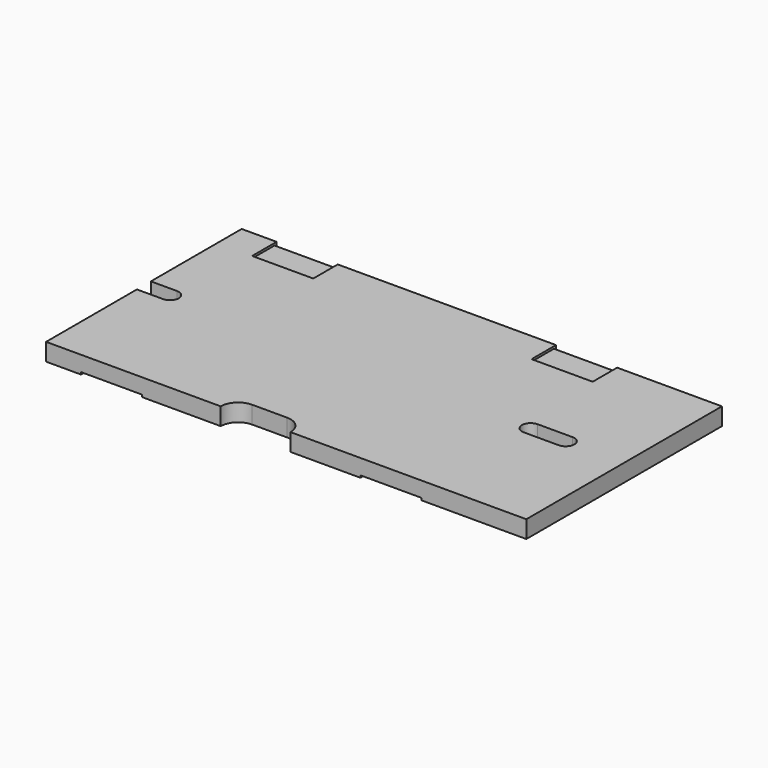
from build123d import *

# Parameters (mm, degrees)
F0_W      = 698.5
F0_H      = 355.6
F1_DEPTH  = 25.4
F2_W      = 88.9
F2_H      = 44.45
F3_DEPTH  = 3.175
F4_W      = 88.9
F4_H      = 44.45
F5_DEPTH  = 3.175
F6_W      = 88.9
F6_H      = 3.81
F7_DEPTH  = 3.175
F8_W      = 88.9
F8_H      = 3.81
F9_DEPTH  = 3.81
F11_DEPTH = 25.4
F12_W     = 101.6
F12_H     = 25.4
F13_DEPTH = 25.4
F14_R     = 25.39999


# Not quite as in the source:
# - a fillet or chamfer is up to 0.001 mm smaller than in the source, because OpenCascade refuses the exact size


with BuildPart() as f1:
    # F0 (on Top) → F1 (new body)
    with BuildSketch(Plane.XY):
        Rectangle(F0_W, F0_H)
    extrude(amount=F1_DEPTH)

    # F2 (on face) → F3 (cut)
    with BuildSketch(Plane.XY.offset(25.4)):
        with Locations((-254, 155.575)):
            Rectangle(F2_W, F2_H)
        with Locations((152.4, 155.575)):
            Rectangle(F2_W, F2_H)
    extrude(amount=-F3_DEPTH, mode=Mode.SUBTRACT)

    # F4 (on face) → F5 (cut)
    with BuildSketch(Plane(origin=(0, 0, 0), x_dir=(1, 0, 0), z_dir=(0, 0, -1))):
        with Locations((-254, 155.575)):
            Rectangle(F4_W, F4_H)
        with Locations((152.4, 155.575)):
            Rectangle(F4_W, F4_H)
    extrude(amount=-F5_DEPTH, mode=Mode.SUBTRACT)

    # F6 (on face) → F7 (cut)
    with BuildSketch(Plane.XY.offset(22.225)):
        with Locations((-254, 175.895)):
            Rectangle(F6_W, F6_H)
    extrude(amount=-F7_DEPTH, mode=Mode.SUBTRACT)

    # F8 (on face) → F9 (cut)
    with BuildSketch(Plane.XY.offset(22.225)):
        with Locations((152.4, 175.895)):
            Rectangle(F8_W, F8_H)
    extrude(amount=-F9_DEPTH, mode=Mode.SUBTRACT)

    # F10 (on face) → F11 (cut)
    with BuildSketch(Plane.XY.offset(25.4)):
        with BuildLine():
            Line((-311.0040204385, -12.7008390054), (-311.0040204385, -12.6991609946))
            ThreePointArc((-311.0040204385, -12.6991609946), (-298.45, 0), (-311.0040204385, 12.6991609946))
            Line((-311.0040204385, 12.6991609946), (-311.2959795615, 12.6991609946))
            Line((-311.2959795615, 12.6991609946), (-354.8822260717, 12.6991609946))
            Line((-354.8822260717, 12.6991609946), (-354.8822260717, -12.7008390054))
            Line((-354.8822260717, -12.7008390054), (-311.0040204385, -12.7008390054))
        make_face()
        with BuildLine():
            Line((-311.2959795615, 12.6991609946), (-311.0040204385, 12.6991609946))
            ThreePointArc((-311.0040204385, 12.6991609946), (-311.15, 12.7), (-311.2959795615, 12.6991609946))
        make_face()
        with BuildLine():
            Line((213.1756003467, 12.7013387805), (213.1756003467, 12.6986612195))
            ThreePointArc((213.1756003467, 12.6986612195), (200.66, 0), (213.1756003467, -12.6986612195))
            Line((213.1756003467, -12.6986612195), (213.5443996533, -12.6986612195))
            Line((213.5443996533, -12.6986612195), (264.16, -12.6986612195))
            ThreePointArc((264.16, -12.6986612195), (276.86, 0.0013387805), (264.16, 12.7013387805))
            Line((264.16, 12.7013387805), (213.1756003467, 12.7013387805))
        make_face()
        with BuildLine():
            Line((213.5443996533, -12.6986612195), (213.1756003467, -12.6986612195))
            ThreePointArc((213.1756003467, -12.6986612195), (213.36, -12.7), (213.5443996533, -12.6986612195))
        make_face()
    extrude(amount=-F11_DEPTH, mode=Mode.SUBTRACT)

    # F12 (on face) → F13 (cut)
    with BuildSketch(Plane.XY.offset(25.4)):
        with Locations((-44.45, -165.1)):
            Rectangle(F12_W, F12_H)
    extrude(amount=-F13_DEPTH, mode=Mode.SUBTRACT)

    # F14 (radius 25.4 in the source; OpenCascade refuses exactly that, so slightly less here)
    f14_edges = [f1.edges().sort_by_distance(p)[0] for p in [
        (-95.25, -152.4, 12.7),
        (6.35, -152.4, 12.7),
    ]]
    fillet(f14_edges, radius=F14_R)


solid = f1.part
